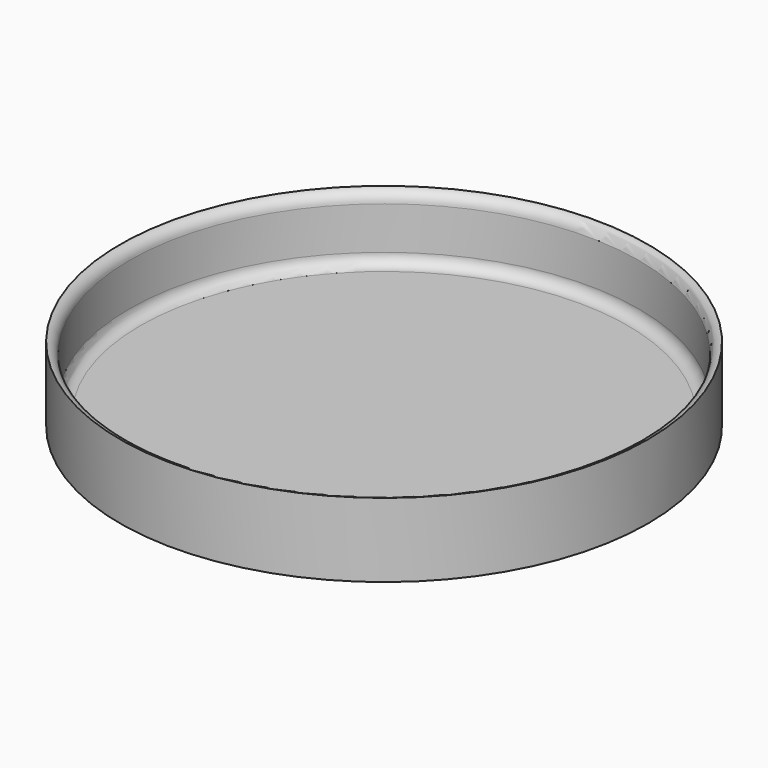
from build123d import *

# Parameters (mm, degrees)
F0_R     = 71.2988650601
F1_DEPTH = 20
F2_T     = -2.5
F3_R     = 3


# Not quite as in the source:
# - a fillet or chamfer that OpenCascade refuses, or shapes differently, is made with other operations: its cross-section is extruded or revolved along the edge and cut away or added


with BuildPart() as f1:
    # F0 (on Top) → F1 (new body)
    with BuildSketch(Plane.XY):
        Circle(F0_R)
    extrude(amount=F1_DEPTH)

    # F2
    f2_openings = [f1.faces().sort_by_distance(p)[0] for p in [
        (0, 0, 20),
    ]]
    offset(amount=F2_T, openings=f2_openings)

    # F3
    f3_edges = [f1.edges().sort_by_distance(p)[0] for p in [
        (-68.798865, 0, 2.5),
    ]]
    fillet(f3_edges, radius=F3_R)

    # F4: fillet of radius 3 on 1 edges, made by hand

    # F4_s1 → F4_t2 (revolve, cut)
    with BuildSketch(Plane.XZ):
        with BuildLine():
            ThreePointArc((68.7988650601, 17.0419601084), (69.5075772126, 18.9784517816), (71.2988650601, 20))
            Line((71.2988650601, 20), (68.7988650601, 20))
            Line((68.7988650601, 20), (68.7988650601, 17.0419601084))
        make_face()
    revolve(axis=Axis((0, 0, 20), (0, 0, 1)), mode=Mode.SUBTRACT)


solid = f1.part
